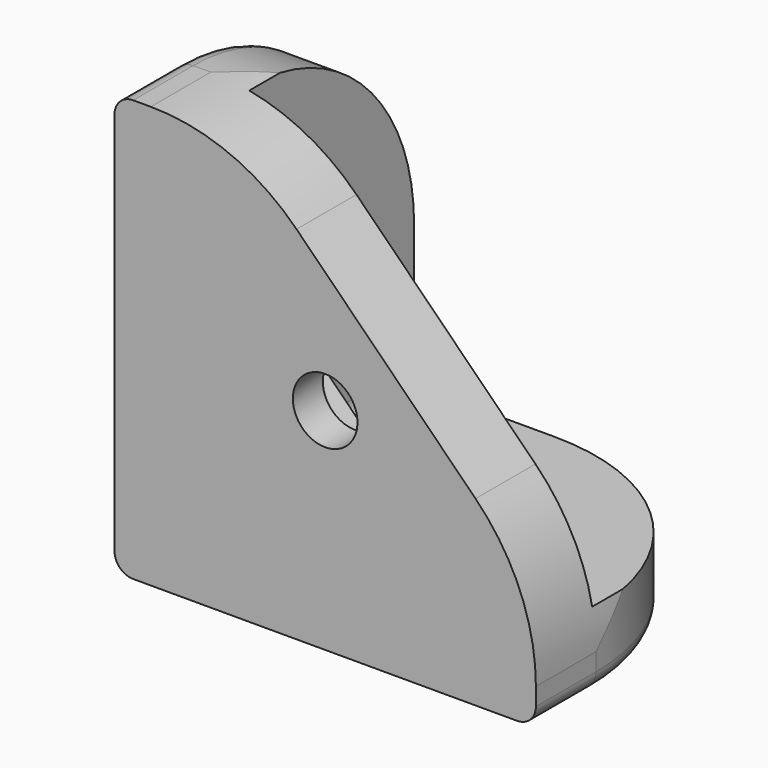
from build123d import *

# Parameters (mm, degrees)
F1_W         = 22.5
F1_H         = 15
F2_DEPTH     = 4
F4_DEPTH     = 18.5
F5_R         = 1.725
F6_DEPTH     = 4
F7_R         = 1.725
F8_DEPTH     = 4
F9_R         = 1.725
F10_DEPTH    = 4
F11_DEPTH    = 2
F12_SIZE     = 16
F13_T1_DEPTH = 59
F13_T3_DEPTH = 59
F13_T5_DEPTH = 26.7817459305
F14_R        = 1


# Not quite as in the source:
# - a fillet or chamfer that OpenCascade refuses, or shapes differently, is made with other operations: its cross-section is extruded or revolved along the edge and cut away or added


with BuildPart() as f2:
    # F1 (on Top) → F2 (new body)
    with BuildSketch(Plane.XY):
        with Locations((11.25, 7.5)):
            Rectangle(F1_W, F1_H)
    extrude(amount=F2_DEPTH)

    # F3 (on face) → F4 (join)
    with BuildSketch(Plane.XY.offset(4)):
        Polygon((4, 15), (0, 15), (0, 0), (22.5, 0), (22.5, 4), (4, 4), align=None)
    extrude(amount=F4_DEPTH)

    # F5 (on face) → F6 (cut, through all)
    with BuildSketch(Plane.XY.offset(4)):
        with Locations((11.25, 7.5)):
            Circle(F5_R)
    extrude(amount=-F6_DEPTH, mode=Mode.SUBTRACT)

    # F7 (on face) → F8 (cut, through all)
    with BuildSketch(Plane.YZ.offset(4)):
        with Locations((7.5, 11.25)):
            Circle(F7_R)
    extrude(amount=-F8_DEPTH, mode=Mode.SUBTRACT)

    # F9 (on face) → F10 (cut, through all)
    with BuildSketch(Plane(origin=(0, 4, 0), x_dir=(-1, 0, 0), z_dir=(0, 1, 0))):
        with Locations((-11.25, 11.25)):
            Circle(F9_R)
    extrude(amount=-F10_DEPTH, mode=Mode.SUBTRACT)

    # F9 (on face) → F11 (cut)
    with BuildSketch(Plane(origin=(0, 4, 0), x_dir=(-1, 0, 0), z_dir=(0, 1, 0))):
        Polygon((-8.1270057994, 10.413196226), (-8.9638095734, 13.5361904266), (-12.086803774, 14.3729942006), (-14.3729942006, 12.086803774), (-13.5361904266, 8.9638095734), (-10.413196226, 8.1270057994), align=None)
        with Locations((-11.25, 11.25)):
            Circle(F9_R, mode=Mode.SUBTRACT)
    extrude(amount=-F11_DEPTH, mode=Mode.SUBTRACT)

    # F12
    f12_edges = [f2.edges().sort_by_distance(p)[0] for p in [
        (22.5, 2, 22.5),
    ]]
    chamfer(f12_edges, length=F12_SIZE)

    # F13: fillet of radius 11 on 4 edges, made by hand

    # F13_s2 → F13_t1 (cut)
    with BuildSketch(Plane.XY.offset(-27.5)):
        with BuildLine():
            ThreePointArc((11.5, 15), (19.2781745931, 11.7781745931), (22.5, 4))
            Line((22.5, 4), (22.5, 15))
            Line((22.5, 15), (11.5, 15))
        make_face()
    extrude(amount=F13_T1_DEPTH, mode=Mode.SUBTRACT)

    # F13_s4 → F13_t3 (cut)
    with BuildSketch(Plane.YZ.offset(-27.5)):
        with BuildLine():
            ThreePointArc((4, 22.5), (11.7781745931, 19.2781745931), (15, 11.5))
            Line((15, 11.5), (15, 22.5))
            Line((15, 22.5), (4, 22.5))
        make_face()
    extrude(amount=F13_T3_DEPTH, mode=Mode.SUBTRACT)

    # F13_s6 → F13_t5 (cut)
    with BuildSketch(Plane.XZ.offset(-15.3908729653)):
        with BuildLine():
            ThreePointArc((1.9436508139, 22.5), (6.1531685699, 21.6626748576), (9.7218254069, 19.2781745931))
            Line((9.7218254069, 19.2781745931), (6.5, 22.5))
            Line((6.5, 22.5), (1.9436508139, 22.5))
        make_face()
        with BuildLine():
            ThreePointArc((19.2781745931, 9.7218254069), (21.6626748576, 6.1531685699), (22.5, 1.9436508139))
            Line((22.5, 1.9436508139), (22.5, 6.5))
            Line((22.5, 6.5), (19.2781745931, 9.7218254069))
        make_face()
    extrude(amount=F13_T5_DEPTH, mode=Mode.SUBTRACT)

    # F14
    f14_edges = [f2.edges().sort_by_distance(p)[0] for p in [
        (0, 2, 22.5),
        (0, 7.5, 0),
        (22.5, 2, 0),
        (4, 9.5, 4),
        (0, 15, 5.75),
        (0, 11.778175, 19.278175),
        (5.75, 15, 0),
        (19.278175, 11.778175, 0),
    ]]
    fillet(f14_edges, radius=F14_R)


solid = f2.part
